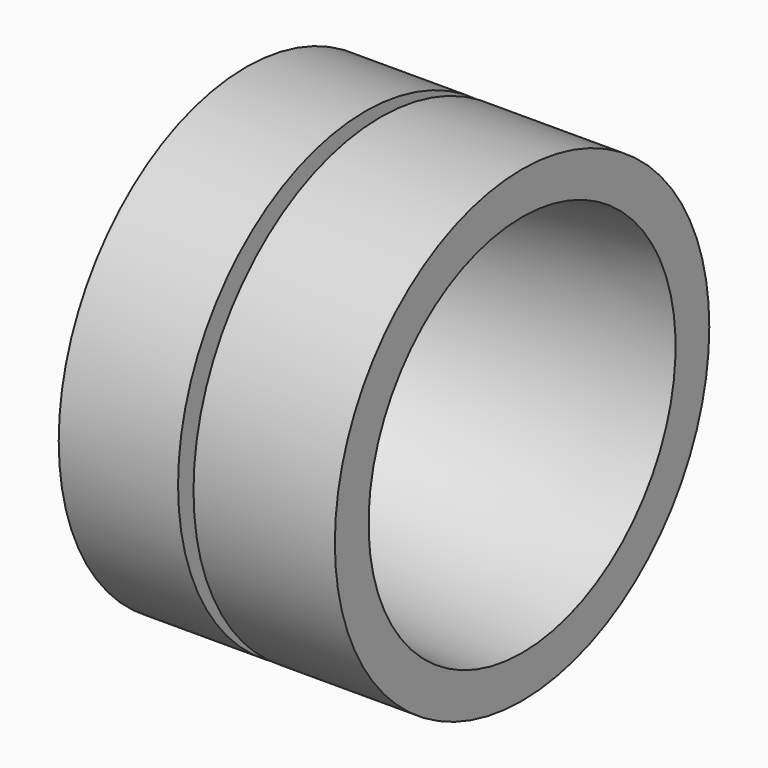
from build123d import *

# Parameters (mm, degrees)
F2_R            = 2.5
F3_DEPTH        = 15
F3_COPIES_COUNT = 3
F4_W            = 3.3
F4_H            = 9.1


# Not quite as in the source:
# - a pattern or mirror of a feature is missing from the dataset's text; its kind, count and spacing are read off the source's solid


with BuildPart() as f1:
    # F0 (on Front) → F1 (revolve)
    with BuildSketch(Plane.XZ):
        with BuildLine():
            Line((59, 50), (0, 50))
            Line((0, 50), (0, 30.5))
            ThreePointArc((0, 30.5), (29.2820901792, 36.97444566), (59, 41))
            Line((59, 41), (59, 50))
        make_face()
    revolve(axis=Axis((-28.7704151153, 0, 0), (-1, 0, 0)))

    # F2 (on face) → F3 (cut)
    with BuildSketch(Plane(origin=(0, 0, 0), x_dir=(0, -1, 0), z_dir=(-1, 0, 0))):
        with Locations((36.8060796608, 21.25)):
            Circle(F2_R)
    f3 = extrude(amount=-F3_DEPTH, mode=Mode.SUBTRACT)

    # F3_copies: F3 ×3 about axis
    f3_copies_axis = Axis((0, 0, 0), (1, 0, 0))
    for i in range(1, F3_COPIES_COUNT):
        add(f3.rotate(f3_copies_axis, i * 360 / F3_COPIES_COUNT), mode=Mode.SUBTRACT)

    # F4 (on Front) → F5 (revolve, cut)
    with BuildSketch(Plane.XZ):
        with Locations((27.15, -45.45)):
            Rectangle(F4_W, F4_H)
    revolve(axis=Axis((25.2881273627, 0, 0), (1, 0, 0)), mode=Mode.SUBTRACT)


solid = f1.part
